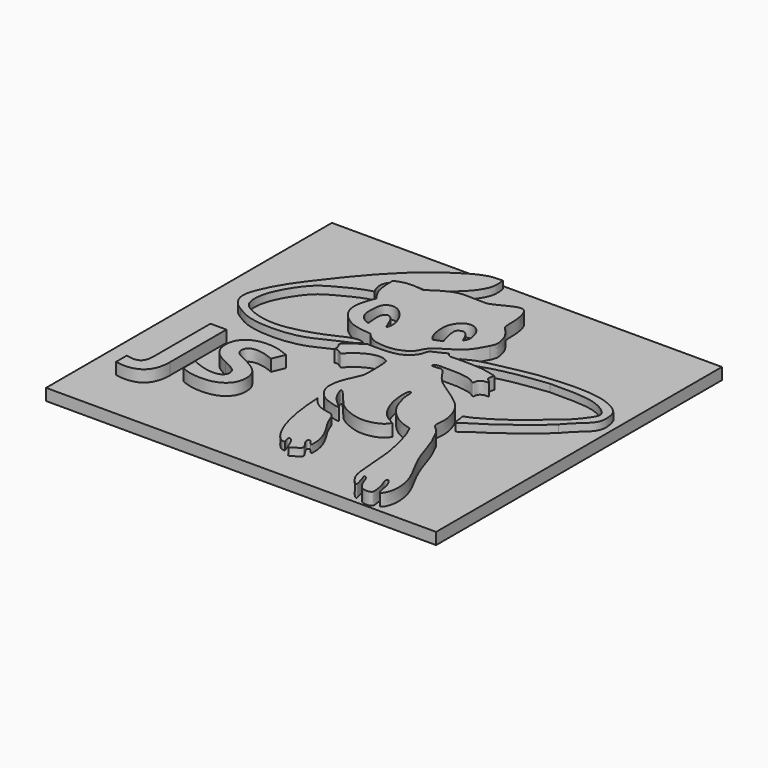
from build123d import *

# Parameters (mm, degrees)
F1_DEPTH     = 5.334
F2_DEPTH     = 3.302
F3_W         = 169.9430719018
F3_H         = 155.6462794542
F4_DEPTH     = 5.08
F5_DEPTH     = 5.08
F6_TEXT_SIZE = 45.9216496286
F7_DEPTH     = 5.08


# Not quite as in the source:
# - Text() gives the source's letters only with a copy of the font that has no kerning and outlines rounded to 1/6400 em; it was checked with that copy


with BuildPart() as f1:
    # F0 (on Top) → F1 (new body)
    with BuildSketch(Plane.XY):
        with BuildLine():
            add(Edge.make_bspline(
                [(-36.8846021593, 36.0807068646), (-37.3919205691, 36.745355779), (-38.573167318, 38.2929329101), (-40.5014475338, 42.4143572996), (-40.7107590613, 48.2182279222), (-40.6138391704, 49.4369952817), (-40.5808985233, 49.8512238264)],
                knots=[0, 0, 0, 0, 0.2194056509, 0.5108669562, 0.8337559114, 1, 1, 1, 1], degree=3))
            add(Edge.make_bspline(
                [(-22.3644245416, 14.6438442171), (-24.6713467296, 14.8439032159), (-29.1783533156, 15.2347561151), (-34.882181479, 17.9727219406), (-39.1312315637, 23.0647945356), (-39.4935763136, 28.8302862551), (-37.8267011281, 33.815991482), (-37.1553457104, 35.4298653868), (-36.8846021593, 36.0807068646)],
                knots=[0, 0, 0, 0, 0.1893684443, 0.3699668893, 0.5515158216, 0.7238806595, 0.8886468645, 1, 1, 1, 1], degree=3))
            add(Edge.make_bspline(
                [(-5.2082133479, 12.2014991939), (-6.1207744444, 11.7172463933), (-8.3286563669, 10.545628396), (-15.353587418, 10.2966075507), (-19.699613734, 11.8971410348), (-21.5102479887, 13.7634179409), (-22.3644245416, 14.6438442171)],
                knots=[0, 0, 0, 0, 0.2165971456, 0.5240426358, 0.775464526, 1, 1, 1, 1], degree=3))
            add(Edge.make_bspline(
                [(15.1303568855, 32.9696908593), (14.5352451306, 31.8316959723), (13.2486953483, 29.3715075085), (10.2455123386, 24.8910940387), (3.5467707647, 21.2909451139), (-0.1632139181, 18.6569829706), (-1.6228436975, 15.6766034686), (-3.1877963332, 12.9531999529), (-4.5795045255, 12.4354117454), (-5.2082133479, 12.2014991939)],
                knots=[0, 0, 0, 0, 0.1407144931, 0.3042053849, 0.4994170574, 0.6491627195, 0.7763538673, 0.8989671128, 1, 1, 1, 1], degree=3))
            add(Edge.make_bspline(
                [(-28.5498145968, 50.8658960462), (-27.3946017427, 51.6630685406), (-24.9466228795, 53.3523342114), (-20.0833499164, 56.0652919109), (-16.3542778469, 56.9634408184), (-12.2867311767, 56.8716252918), (-6.9153223537, 56.7342359886), (-4.3946916269, 56.665054576), (1.0627636823, 59.6982249817), (4.5886739884, 61.236413898), (8.2470343675, 61.4891197316), (9.8575595266, 56.0097175618), (10.1904654801, 52.4142595185), (10.0843781414, 47.0754303269), (11.5893851176, 45.8127835913), (14.8613176101, 41.8496715208), (15.5576528197, 39.0147495294), (16.4135900587, 35.7580508966), (15.5545549064, 33.8914382347), (15.1303568855, 32.9696908593)],
                knots=[0, 0, 0, 0, 0.0621112649, 0.1316182234, 0.188871196, 0.2491962953, 0.3167553376, 0.3643401957, 0.436758445, 0.4967888689, 0.546791506, 0.6123099758, 0.6728165948, 0.7378250462, 0.7790399568, 0.8445049968, 0.8965058511, 0.9488938107, 1, 1, 1, 1], degree=3))
            add(Edge.make_bspline(
                [(-40.5808985233, 49.8512238264), (-39.7577733728, 50.1889108848), (-38.0437485114, 50.8920895121), (-34.9342862767, 51.5058179945), (-31.3792002355, 51.3783823788), (-29.458277106, 51.0304457679), (-28.5498145968, 50.8658960462)],
                knots=[0, 0, 0, 0, 0.234957575, 0.4892611102, 0.7584561682, 1, 1, 1, 1], degree=3))
        make_face()
        with BuildLine():
            add(Edge.make_bspline(
                [(-27.7441535145, 20.2597975731), (-27.836523165, 21.3377254697), (-28.0205851584, 23.4856772729), (-28.2064858053, 26.7533419634), (-27.3095138698, 28.5803581568), (-25.8242693753, 29.158776732), (-23.9397520395, 27.8647529376), (-22.7818146955, 25.7716562911), (-21.7167721967, 22.9536226595), (-21.1669852724, 21.9621876443), (-20.9360662848, 21.5457696468)],
                knots=[0, 0, 0, 0, 0.1498442019, 0.2985896596, 0.4110847443, 0.5056814579, 0.6233821967, 0.7537217582, 0.89655934, 1, 1, 1, 1], degree=3))
            add(Edge.make_bspline(
                [(-20.9360662848, 21.5457696468), (-20.6845803928, 22.4517973521), (-20.1286034759, 24.4548142458), (-21.2599441765, 28.7542103146), (-23.5058865444, 32.3709839432), (-26.9334066004, 35.3160516517), (-30.5123126311, 35.2735079139), (-32.7990191763, 33.0795235548), (-32.9444978647, 29.4825750713), (-33.2245472294, 25.7467879432), (-31.8503260445, 22.5933797005), (-29.5656235756, 20.8892744088), (-28.312173584, 20.4560980688), (-27.7441535145, 20.2597975731)],
                knots=[0, 0, 0, 0, 0.0851228406, 0.1881868366, 0.292340602, 0.3959368999, 0.4853122137, 0.5684365665, 0.6615536453, 0.7584972412, 0.8490847261, 0.9316104312, 1, 1, 1, 1], degree=3))
        make_face(mode=Mode.SUBTRACT)
        with BuildLine():
            add(Edge.make_bspline(
                [(5.4089953192, 30.3651615977), (4.9974793972, 31.3635089709), (4.2164206085, 33.2583760916), (2.492858238, 35.4574563274), (1.1828097347, 35.7536675932), (-1.0889632523, 34.9032052933), (-1.0761434624, 32.5663825666), (-0.7105408655, 30.3909840554), (-0.0619549295, 27.5454399373), (0.4242136144, 26.3185378529), (0.6415589014, 25.7700420916)],
                knots=[0, 0, 0, 0, 0.1500445323, 0.2847850944, 0.377641595, 0.497182947, 0.616278328, 0.7433829902, 0.8852774448, 1, 1, 1, 1], degree=3))
            Line((0.6415589014, 25.7700420916), (-3.0919760466, 24.3340656161))
            add(Edge.make_bspline(
                [(-3.0919760466, 24.3340656161), (-3.6746172439, 25.0952157056), (-4.9790959932, 26.7993590469), (-5.9269204187, 31.3877090281), (-5.8129309399, 36.1864843136), (-3.2806174064, 39.831657957), (-1.0494876922, 41.0503171402), (2.1831388461, 41.2713590695), (5.273039036, 38.380179271), (6.3476776556, 34.9097936113), (6.6819460197, 32.0494739818), (5.8108081984, 30.8968227282), (5.4089953192, 30.3651615977)],
                knots=[0, 0, 0, 0, 0.0943242152, 0.2111830315, 0.3310976043, 0.4422336843, 0.5274260332, 0.6207101402, 0.729021317, 0.8337202238, 0.9233033465, 1, 1, 1, 1], degree=3))
        make_face(mode=Mode.SUBTRACT)
    extrude(amount=F1_DEPTH)


with BuildPart() as f1b:
    # F0 (on Top) → F1, piece 2 (new body)
    with BuildSketch(Plane.XY):
        with BuildLine():
            add(Edge.make_bspline(
                [(30.0683174282, 16.6960265487), (27.7743567444, 17.2982553033), (22.996366427, 18.5526112206), (14.1217566151, 18.5069548483), (10.9595550033, 18.4055071495), (8.914888562, 18.2892193751), (8.1286790312, 19.3965578852), (7.7262688428, 19.9633333832)],
                knots=[0, 0, 0, 0, 0.2687230853, 0.5597115543, 0.7341470669, 0.8639269499, 1, 1, 1, 1], degree=3))
            add(Edge.make_bspline(
                [(7.7262688428, 19.9633333832), (6.7843841918, 19.4219987594), (4.8626373132, 18.3175024471), (0.9491517041, 16.983214183), (0.9172062675, 14.0816922981), (-1.1563972414, 11.1645043961), (-4.2681909188, 8.7975654115), (-10.2481427233, 7.7101704983), (-15.7637806819, 7.8784264398), (-17.5742383687, 7.9638167156), (-18.2920843363, 7.9976739362)],
                knots=[0, 0, 0, 0, 0.1189762035, 0.2427496271, 0.3446266716, 0.463365679, 0.5892044553, 0.7483578638, 0.9002239632, 1, 1, 1, 1], degree=3))
            add(Edge.make_bspline(
                [(-18.2920843363, 7.9976739362), (-19.2081909322, 7.3508545619), (-21.220968544, 5.9297278487), (-26.2844384077, 2.5837754081), (-25.5818429798, 1.1641009834), (-24.788360107, 0.7943681377), (-24.7400624967, -0.7928668879), (-24.7462409395, -1.4706101124), (-24.7490536422, -1.7791490536)],
                knots=[0, 0, 0, 0, 0.2335516694, 0.5131363244, 0.6318283516, 0.7367278182, 0.8801467617, 1, 1, 1, 1], degree=3))
            add(Edge.make_bspline(
                [(-24.7490536422, -1.7791490536), (-24.2594300604, -1.6489843167), (-23.1371940302, -1.3506417469), (-20.7418558435, -3.9319628807), (-19.8396284785, -1.3153314822), (-15.2791573927, 1.747858691), (-12.0049756273, 3.1979621252), (-8.2035408147, 3.7607412239), (-6.3214470372, 2.7044753683), (-5.4122591391, 2.1942222957)],
                knots=[0, 0, 0, 0, 0.1027998361, 0.2356211674, 0.3469371625, 0.5398555958, 0.7001501422, 0.8551507554, 1, 1, 1, 1], degree=3))
            add(Edge.make_bspline(
                [(-5.4122591391, -11.4604206756), (-5.2622117063, -11.0833952824), (-4.8483954868, -10.0435959346), (-4.8531432648, -5.796717989), (-4.8905091249, -0.455510217), (-5.2613557919, 1.4278523975), (-5.4122591391, 2.1942222957)],
                knots=[0, 0, 0, 0, 0.16298087, 0.4494853805, 0.7759869344, 1, 1, 1, 1], degree=3))
            add(Edge.make_bspline(
                [(-5.4122591391, -11.4604206756), (-5.7180365241, -12.1910633261), (-6.4589745929, -13.9615047682), (-8.7341618296, -18.823732403), (-9.3339817846, -22.6702412315), (-9.3862087635, -25.4827799286), (-8.6161951623, -27.2256408895), (-8.2267019898, -28.1072258949)],
                knots=[0, 0, 0, 0, 0.1760181488, 0.4265146922, 0.6415927054, 0.8187081449, 1, 1, 1, 1], degree=3))
            add(Edge.make_bspline(
                [(-8.2267019898, -28.1072258949), (-7.6234509095, -28.9847780463), (-6.3158368471, -30.886970303), (-3.3578440432, -33.0385452557), (4.7605685311, -35.3009211391), (0.7062696421, -32.348079143), (-2.6369370543, -28.938166705), (-4.7745965374, -23.008879984), (-2.1692361288, -25.4214104232), (0.0596427785, -28.1204059957), (3.5703763797, -32.828689266), (9.4441591128, -35.6788887604), (15.6783436568, -37.2193911759), (22.840726257, -35.0789922839), (24.1300062291, -32.9878270093), (24.6503651142, -32.1438238025)],
                knots=[0, 0, 0, 0, 0.0644771481, 0.1397614166, 0.2278212025, 0.2838940026, 0.3731896446, 0.4478304981, 0.4963143315, 0.5679076052, 0.6548180235, 0.7466462144, 0.8393730298, 0.9351702711, 1, 1, 1, 1], degree=3))
            add(Edge.make_bspline(
                [(24.6503651142, -32.1438238025), (22.7874017729, -31.1547850766), (18.978892069, -29.1328646762), (15.7565133464, -22.5588668197), (14.3110475227, -17.0219112758), (14.2258983476, -9.955668629), (16.1051306441, -10.5144580218), (15.6702473707, -13.747750159), (17.0855807883, -18.568062254), (18.3355817835, -22.1596484216), (21.6146077655, -26.502386498), (26.1560860605, -29.9186464967), (29.8500456849, -30.9730548373), (31.7023843527, -31.501788646)],
                knots=[0, 0, 0, 0, 0.1044502141, 0.213530586, 0.3203453584, 0.4213187613, 0.4580269744, 0.5290816996, 0.6236498562, 0.7054940824, 0.8011178875, 0.9002704239, 1, 1, 1, 1], degree=3))
            add(Edge.make_bspline(
                [(31.7023843527, -31.501788646), (32.4317515175, -33.0339186757), (34.0418847304, -36.4162116639), (35.891222752, -44.0199699231), (36.7066142268, -48.1595329342), (36.9354538826, -49.5206387254), (37.0256751776, -50.0572621822)],
                knots=[0, 0, 0, 0, 0.2736015544, 0.6039961368, 0.8438732953, 1, 1, 1, 1], degree=3))
            add(Edge.make_bspline(
                [(37.0256751776, -50.0572621822), (37.2529570378, -52.2585996466), (37.7295250837, -56.874397374), (38.1744288141, -65.147375762), (39.0614282703, -71.473936135), (43.7073747885, -75.9926535392), (43.0041439625, -73.1870722683), (42.5863736095, -71.2442159702), (41.2192631142, -68.0900104475), (43.2122596535, -69.062811459), (43.8660534195, -72.1091856839), (46.0001837404, -75.8667367907), (48.2415322815, -76.7510536361), (51.5666329574, -76.464046498), (51.0718324014, -73.597450229), (50.7537782092, -69.9651897279), (49.0133489818, -67.3461961901), (49.5300726584, -65.1991280143), (51.3610203699, -67.2721869465), (52.3453968623, -70.4529473283), (52.995619021, -76.2204950553), (56.059449066, -71.996615036), (56.1941191956, -64.2541648711), (53.057015864, -56.2370554706), (47.5422537848, -47.2864849217), (44.2428025956, -35.181683009), (42.4634124655, -31.9627538165), (41.779063642, -30.7247620076)],
                knots=[0, 0, 0, 0, 0.0515181447, 0.1080240258, 0.1600193281, 0.200966199, 0.2242692528, 0.2561913518, 0.2869292175, 0.3071601688, 0.3426397052, 0.3829711635, 0.4133879878, 0.44506026, 0.4747807776, 0.5132716918, 0.5483859123, 0.5705941331, 0.5969574393, 0.6366393869, 0.6760617143, 0.7097084145, 0.7649651301, 0.8224062602, 0.8873011559, 0.9566563172, 1, 1, 1, 1], degree=3))
            add(Edge.make_bspline(
                [(41.779063642, -30.7247620076), (41.220519955, -29.4131194944), (40.1405083976, -26.8769005623), (36.3496730282, -24.6391556022), (37.9091307315, -19.6176807334), (35.5635143336, -10.6479929739), (30.5388392719, -5.8669855098), (23.9637593307, -1.3236326178), (17.1210038146, 2.9501551711), (13.8645399549, 9.8095100123), (11.3218741684, 9.2331700055), (8.0189997491, 8.9048258219), (9.6884536448, 10.9398859033), (12.9400373278, 10.6519892488), (17.7385160156, 10.8919830294), (21.7909115084, 10.3524706804), (25.1173197763, 9.8387273821), (27.8544362389, 7.7039501469), (27.5140398783, 10.0552824679), (29.4509197324, 11.6524955754), (32.6539040013, 11.3234634506), (30.9452406108, 12.542717614), (30.0683174282, 13.1684653461)],
                knots=[0, 0, 0, 0, 0.0519267935, 0.1004067156, 0.1547860225, 0.2308120849, 0.2975658467, 0.3688932812, 0.4426002883, 0.5078563984, 0.5467057553, 0.5855180915, 0.6152135834, 0.6611250141, 0.7174470552, 0.7689076739, 0.8172224822, 0.8564603738, 0.8862383123, 0.9262880687, 0.962169435, 1, 1, 1, 1], degree=3))
            add(Edge.make_bspline(
                [(30.0683174282, 13.1684653461), (29.9041852058, 13.3684306238), (29.4381629957, 13.9361939752), (29.8205842702, 15.6110511778), (30.0683174282, 16.6960265487)],
                knots=[0, 0, 0, 0, 0.3521982834, 1, 1, 1, 1], degree=3))
        make_face()
    extrude(amount=F1_DEPTH)


with BuildPart() as f2:
    # F0 (on Top) → F2 (new body)
    with BuildSketch(Plane.XY):
        with BuildLine():
            add(Edge.make_bspline(
                [(-43.0377721786, 42.7853837609), (-43.4217519294, 43.5555106027), (-44.2704707094, 45.2577386818), (-44.7495303082, 49.6843935754), (-41.0137641329, 52.7815034964), (-36.6859509281, 54.4525017318), (-31.3441059726, 54.4142323895), (-29.2217337248, 54.0177284331), (-28.3044036478, 53.8463518023)],
                knots=[0, 0, 0, 0, 0.1383428068, 0.3057821096, 0.4812834692, 0.6632360629, 0.8544441539, 1, 1, 1, 1], degree=3))
            add(Edge.make_bspline(
                [(-28.3044036478, 53.8463518023), (-26.4073160355, 55.6555092544), (-22.6771829073, 59.2127504184), (-17.2353435255, 63.8393788129), (-13.8276032853, 69.6509731284), (-13.5447997553, 73.3805690433), (-13.8346112059, 75.3733824514), (-13.9714321122, 76.3141959906)],
                knots=[0, 0, 0, 0, 0.2399087284, 0.471718591, 0.6909669262, 0.8541045044, 1, 1, 1, 1], degree=3))
            add(Edge.make_bspline(
                [(-13.9714321122, 76.3141959906), (-15.6695767931, 76.3303285057), (-19.2883266624, 76.3647069291), (-25.3938334761, 73.7499379423), (-32.2227465198, 69.3257394868), (-37.0027510136, 65.6788461869), (-41.5089383745, 61.9702597728), (-43.2950078592, 60.2558688539), (-44.0782904625, 59.5040209591)],
                knots=[0, 0, 0, 0, 0.1571726677, 0.3349352838, 0.5326783847, 0.7051580212, 0.870696748, 1, 1, 1, 1], degree=3))
            add(Edge.make_bspline(
                [(-44.0782904625, 59.5040209591), (-46.5278412391, 57.082066591), (-52.097162839, 51.575488444), (-63.3309865981, 37.4942248425), (-71.4221468374, 26.4624379543), (-75.7339498561, 17.0106297705), (-76.6395144361, 11.8788318896), (-75.1074330935, 8.3160305556), (-73.204783322, 6.068043111), (-71.7088671371, 5.0905988199), (-70.9798410535, 4.6142470092)],
                knots=[0, 0, 0, 0, 0.1518529739, 0.3452543444, 0.517129726, 0.6613859031, 0.7623466126, 0.8489157512, 0.9263699669, 1, 1, 1, 1], degree=3))
            add(Edge.make_bspline(
                [(-70.9798410535, 4.6142470092), (-69.3666307118, 3.5770845145), (-65.6901376032, 1.2133997143), (-55.8893542983, -0.5183749), (-41.2432784113, 0.4464145968), (-31.0706871572, 6.483604405), (-24.0806480786, 8.8396956503), (-21.752412637, 11.3394508322), (-26.5347743619, 12.1529097756), (-32.3033005496, 9.1331545972), (-40.0565385081, 5.9205974959), (-50.0430210503, 3.1697487317), (-58.8129954214, 2.9178477888), (-66.9351159188, 5.4707126725), (-72.0186295298, 9.156570048), (-71.6690554507, 18.4329778003), (-66.5327096092, 27.8683616368), (-61.2862876559, 34.4220241119), (-54.7268271319, 37.7283730842), (-48.6744931046, 41.0395084453), (-44.8645902562, 42.2195589437), (-43.0377721786, 42.7853837609)],
                knots=[0, 0, 0, 0, 0.0465524502, 0.1060926513, 0.1790243597, 0.2452061951, 0.2968084881, 0.3232171179, 0.357646466, 0.4069920351, 0.4626730308, 0.5238603294, 0.5805035455, 0.6354123547, 0.6802029703, 0.7351769542, 0.7981924539, 0.8529702112, 0.9040331392, 0.9539846544, 1, 1, 1, 1], degree=3))
        make_face()
    extrude(amount=F2_DEPTH)


with BuildPart() as f2b:
    # F0 (on Top) → F2, piece 2 (new body)
    with BuildSketch(Plane.XY):
        with BuildLine():
            add(Edge.make_bspline(
                [(2.3568598554, -62.7967566252), (1.849591697, -62.7900183143), (0.4679465245, -62.7716651917), (-3.2310828631, -58.8113433278), (-6.7057614708, -50.0665204215), (-8.6370836456, -38.8411168477), (-8.9614558541, -33.2628901217), (-9.1090472415, -30.7247620076)],
                knots=[0, 0, 0, 0, 0.099509161, 0.2710328838, 0.51388907, 0.7788164808, 1, 1, 1, 1], degree=3))
            add(Edge.make_bspline(
                [(-9.1090472415, -30.7247620076), (-8.4235955574, -31.6189211927), (-6.9475052353, -33.5444540203), (-3.101528472, -36.1875069597), (1.8982272323, -36.366099626), (3.4405558722, -38.6877901024), (4.4761606927, -42.3593420867), (7.8964967826, -47.1650437774), (10.103858215, -52.0425869753), (10.7860608645, -55.6476684863), (10.6753618785, -57.5461375395), (10.9225050319, -59.3049638311), (9.4107167153, -57.6424469164), (8.5616404275, -56.4503239427), (7.5237963592, -56.8148042208), (7.6117730332, -58.1583165289), (8.9359028975, -60.1929547878), (10.1219675513, -61.7535687362), (9.4773292634, -62.9623853428), (7.0627564007, -64.3325582518), (5.4694748144, -65.4986569004), (4.5573424059, -62.78355908), (3.3761804254, -60.4551449839), (2.1377112045, -59.3756823228), (1.4345728768, -60.1256467658), (1.8841051195, -61.4401596052), (2.1958233582, -62.3346530955), (2.3568598554, -62.7967566252)],
                knots=[0, 0, 0, 0, 0.0496809561, 0.1069857733, 0.1646060762, 0.2058387605, 0.2571628324, 0.3222353289, 0.3845712685, 0.4346179158, 0.4726711954, 0.4992092936, 0.5325676268, 0.5654673868, 0.5880449987, 0.6160765379, 0.6586074123, 0.6943476006, 0.72222254, 0.7675356615, 0.7994953394, 0.8396297218, 0.8851573032, 0.9154600181, 0.9370908196, 0.9675005412, 1, 1, 1, 1], degree=3))
        make_face()
    extrude(amount=F2_DEPTH)


with BuildPart() as f2c:
    # F0 (on Top) → F2, piece 3 (new body)
    with BuildSketch(Plane.XY):
        with BuildLine():
            add(Edge.make_bspline(
                [(10.7216527686, 22.0162756741), (12.1246687267, 22.8148610446), (15.339687331, 24.6448237106), (23.6197362006, 26.4763189676), (32.72292454, 28.3516074967), (37.0192507628, 29.0816873989), (38.9400422573, 29.4080898166)],
                knots=[0, 0, 0, 0, 0.210423914, 0.4821875291, 0.7684976098, 1, 1, 1, 1], degree=3))
            add(Edge.make_bspline(
                [(10.7216527686, 22.0162756741), (11.0952281861, 21.6401005628), (11.9676852339, 20.7615721278), (15.1851161792, 20.2060896425), (20.1867499974, 22.1900920896), (27.3159099422, 24.2389696372), (36.615664636, 25.8884813304), (42.8756191809, 26.6520064029), (46.0081286728, 27.0340777934)],
                knots=[0, 0, 0, 0, 0.0904593315, 0.2112609063, 0.3729533578, 0.5659140772, 0.7827814461, 1, 1, 1, 1], degree=3))
            add(Edge.make_bspline(
                [(46.0081286728, 27.0340777934), (48.7258841079, 27.0612678355), (54.4256706903, 27.1182918912), (64.5466285691, 26.6819854244), (71.2784960569, 23.5683344076), (74.4956568823, 20.0928312055), (72.370302212, 16.1583995878), (68.2328509473, 10.8727360954), (63.0282482519, 6.6939099868), (60.288196872, 4.4211072069), (59.0115785599, 3.3621848561)],
                knots=[0, 0, 0, 0, 0.1437483771, 0.3014749084, 0.4359008913, 0.5332154076, 0.6294905174, 0.7592457502, 0.8878301019, 1, 1, 1, 1], degree=3))
            add(Edge.make_bspline(
                [(59.0115785599, 3.3621848561), (56.9423383347, 1.6375621217), (52.775286197, -1.8354966196), (46.5278179073, -6.1349616625), (39.331175356, -10.0891007633), (37.5946538004, -10.0778540145), (38.361869053, -11.9948167923), (38.4145231293, -16.8707660308), (41.9490027911, -13.083803004), (47.7757044759, -10.0981764978), (54.0702257822, -5.0810900312), (60.5319653238, -0.5910086566), (64.8441388463, 3.4273348996), (67.067630589, 5.4993187077)],
                knots=[0, 0, 0, 0, 0.1094389502, 0.2203890133, 0.3295663194, 0.369726266, 0.4213415268, 0.4936271411, 0.5627007536, 0.6656686645, 0.7754420094, 0.884210866, 1, 1, 1, 1], degree=3))
            add(Edge.make_bspline(
                [(67.067630589, 5.4993187077), (68.4073962182, 7.0026565142), (71.2661439341, 10.3161375403), (78.3602736598, 15.59597471), (76.7631828785, 22.33495377), (75.9328380227, 24.1133533418)],
                knots=[0, 0, 0, 0, 0.3098887474, 0.6604961476, 1, 1, 1, 1], degree=3))
            add(Edge.make_bspline(
                [(38.9400422573, 29.4080898166), (42.1234440462, 29.7199891996), (48.5724313187, 30.3518400576), (58.6475201749, 30.6661036157), (67.9584350083, 29.3917039016), (73.8641097497, 26.3531807622), (75.3402605954, 24.7549413105), (75.9328380227, 24.1133533418)],
                knots=[0, 0, 0, 0, 0.2286564396, 0.4632159453, 0.6902384315, 0.8756511139, 1, 1, 1, 1], degree=3))
        make_face()
    extrude(amount=F2_DEPTH)


with BuildPart() as f4:
    # F3 (on face) → F4 (new body)
    with BuildSketch(Plane(origin=(0, 0, 0), x_dir=(1, 0, 0), z_dir=(0, 0, -1))):
        with Locations((-4.9392692745, -0.3463253379)):
            Rectangle(F3_W, F3_H)
        with BuildLine():
            add(Edge.make_bspline(
                [(30.0683174282, -13.1684653461), (29.9041852058, -13.3684306238), (29.4381629957, -13.9361939752), (29.8205842702, -15.6110511778), (30.0683174282, -16.6960265487)],
                knots=[0, 0, 0, 0, 0.3521982834, 1, 1, 1, 1], degree=3))
            add(Edge.make_bspline(
                [(30.0683174282, -16.6960265487), (27.7743567444, -17.2982553033), (22.996366427, -18.5526112206), (14.1217566151, -18.5069548483), (10.9595550033, -18.4055071495), (8.914888562, -18.2892193751), (8.1286790312, -19.3965578852), (7.7262688428, -19.9633333832)],
                knots=[0, 0, 0, 0, 0.2687230853, 0.5597115543, 0.7341470669, 0.8639269499, 1, 1, 1, 1], degree=3))
            add(Edge.make_bspline(
                [(7.7262688428, -19.9633333832), (6.7843841918, -19.4219987594), (4.8626373132, -18.3175024471), (0.9491517041, -16.983214183), (0.9172062675, -14.0816922981), (-1.1563972414, -11.1645043961), (-4.2681909188, -8.7975654115), (-10.2481427233, -7.7101704983), (-15.7637806819, -7.8784264398), (-17.5742383687, -7.9638167156), (-18.2920843363, -7.9976739362)],
                knots=[0, 0, 0, 0, 0.1189762035, 0.2427496271, 0.3446266716, 0.463365679, 0.5892044553, 0.7483578638, 0.9002239632, 1, 1, 1, 1], degree=3))
            add(Edge.make_bspline(
                [(-18.2920843363, -7.9976739362), (-19.2081909322, -7.3508545619), (-21.220968544, -5.9297278487), (-26.2844384077, -2.5837754081), (-25.5818429798, -1.1641009834), (-24.788360107, -0.7943681377), (-24.7400624967, 0.7928668879), (-24.7462409395, 1.4706101124), (-24.7490536422, 1.7791490536)],
                knots=[0, 0, 0, 0, 0.2335516694, 0.5131363244, 0.6318283516, 0.7367278182, 0.8801467617, 1, 1, 1, 1], degree=3))
            add(Edge.make_bspline(
                [(-24.7490536422, 1.7791490536), (-24.2594300604, 1.6489843167), (-23.1371940302, 1.3506417469), (-20.7418558435, 3.9319628807), (-19.8396284785, 1.3153314822), (-15.2791573927, -1.747858691), (-12.0049756273, -3.1979621252), (-8.2035408147, -3.7607412239), (-6.3214470372, -2.7044753683), (-5.4122591391, -2.1942222957)],
                knots=[0, 0, 0, 0, 0.1027998361, 0.2356211674, 0.3469371625, 0.5398555958, 0.7001501422, 0.8551507554, 1, 1, 1, 1], degree=3))
            add(Edge.make_bspline(
                [(-5.4122591391, 11.4604206756), (-5.2622117063, 11.0833952824), (-4.8483954868, 10.0435959346), (-4.8531432648, 5.796717989), (-4.8905091249, 0.455510217), (-5.2613557919, -1.4278523975), (-5.4122591391, -2.1942222957)],
                knots=[0, 0, 0, 0, 0.16298087, 0.4494853805, 0.7759869344, 1, 1, 1, 1], degree=3))
            add(Edge.make_bspline(
                [(-5.4122591391, 11.4604206756), (-5.7180365241, 12.1910633261), (-6.4589745929, 13.9615047682), (-8.7341618296, 18.823732403), (-9.3339817846, 22.6702412315), (-9.3862087635, 25.4827799286), (-8.6161951623, 27.2256408895), (-8.2267019898, 28.1072258949)],
                knots=[0, 0, 0, 0, 0.1760181488, 0.4265146922, 0.6415927054, 0.8187081449, 1, 1, 1, 1], degree=3))
            add(Edge.make_bspline(
                [(-8.2267019898, 28.1072258949), (-7.6234509095, 28.9847780463), (-6.3158368471, 30.886970303), (-3.3578440432, 33.0385452557), (4.7605685311, 35.3009211391), (0.7062696421, 32.348079143), (-2.6369370543, 28.938166705), (-4.7745965374, 23.008879984), (-2.1692361288, 25.4214104232), (0.0596427785, 28.1204059957), (3.5703763797, 32.828689266), (9.4441591128, 35.6788887604), (15.6783436568, 37.2193911759), (22.840726257, 35.0789922839), (24.1300062291, 32.9878270093), (24.6503651142, 32.1438238025)],
                knots=[0, 0, 0, 0, 0.0644771481, 0.1397614166, 0.2278212025, 0.2838940026, 0.3731896446, 0.4478304981, 0.4963143315, 0.5679076052, 0.6548180235, 0.7466462144, 0.8393730298, 0.9351702711, 1, 1, 1, 1], degree=3))
            add(Edge.make_bspline(
                [(24.6503651142, 32.1438238025), (22.7874017729, 31.1547850766), (18.978892069, 29.1328646762), (15.7565133464, 22.5588668197), (14.3110475227, 17.0219112758), (14.2258983476, 9.955668629), (16.1051306441, 10.5144580218), (15.6702473707, 13.747750159), (17.0855807883, 18.568062254), (18.3355817835, 22.1596484216), (21.6146077655, 26.502386498), (26.1560860605, 29.9186464967), (29.8500456849, 30.9730548373), (31.7023843527, 31.501788646)],
                knots=[0, 0, 0, 0, 0.1044502141, 0.213530586, 0.3203453584, 0.4213187613, 0.4580269744, 0.5290816996, 0.6236498562, 0.7054940824, 0.8011178875, 0.9002704239, 1, 1, 1, 1], degree=3))
            add(Edge.make_bspline(
                [(31.7023843527, 31.501788646), (32.4317515175, 33.0339186757), (34.0418847304, 36.4162116639), (35.891222752, 44.0199699231), (36.7066142268, 48.1595329342), (36.9354538826, 49.5206387254), (37.0256751776, 50.0572621822)],
                knots=[0, 0, 0, 0, 0.2736015544, 0.6039961368, 0.8438732953, 1, 1, 1, 1], degree=3))
            add(Edge.make_bspline(
                [(37.0256751776, 50.0572621822), (37.2529570378, 52.2585996466), (37.7295250837, 56.874397374), (38.1744288141, 65.147375762), (39.0614282703, 71.473936135), (43.7073747885, 75.9926535392), (43.0041439625, 73.1870722683), (42.5863736095, 71.2442159702), (41.2192631142, 68.0900104475), (43.2122596535, 69.062811459), (43.8660534195, 72.1091856839), (46.0001837404, 75.8667367907), (48.2415322815, 76.7510536361), (51.5666329574, 76.464046498), (51.0718324014, 73.597450229), (50.7537782092, 69.9651897279), (49.0133489818, 67.3461961901), (49.5300726584, 65.1991280143), (51.3610203699, 67.2721869465), (52.3453968623, 70.4529473283), (52.995619021, 76.2204950553), (56.059449066, 71.996615036), (56.1941191956, 64.2541648711), (53.057015864, 56.2370554706), (47.5422537848, 47.2864849217), (44.2428025956, 35.181683009), (42.4634124655, 31.9627538165), (41.779063642, 30.7247620076)],
                knots=[0, 0, 0, 0, 0.0515181447, 0.1080240258, 0.1600193281, 0.200966199, 0.2242692528, 0.2561913518, 0.2869292175, 0.3071601688, 0.3426397052, 0.3829711635, 0.4133879878, 0.44506026, 0.4747807776, 0.5132716918, 0.5483859123, 0.5705941331, 0.5969574393, 0.6366393869, 0.6760617143, 0.7097084145, 0.7649651301, 0.8224062602, 0.8873011559, 0.9566563172, 1, 1, 1, 1], degree=3))
            add(Edge.make_bspline(
                [(41.779063642, 30.7247620076), (41.220519955, 29.4131194944), (40.1405083976, 26.8769005623), (36.3496730282, 24.6391556022), (37.9091307315, 19.6176807334), (35.5635143336, 10.6479929739), (30.5388392719, 5.8669855098), (23.9637593307, 1.3236326178), (17.1210038146, -2.9501551711), (13.8645399549, -9.8095100123), (11.3218741684, -9.2331700055), (8.0189997491, -8.9048258219), (9.6884536448, -10.9398859033), (12.9400373278, -10.6519892488), (17.7385160156, -10.8919830294), (21.7909115084, -10.3524706804), (25.1173197763, -9.8387273821), (27.8544362389, -7.7039501469), (27.5140398783, -10.0552824679), (29.4509197324, -11.6524955754), (32.6539040013, -11.3234634506), (30.9452406108, -12.542717614), (30.0683174282, -13.1684653461)],
                knots=[0, 0, 0, 0, 0.0519267935, 0.1004067156, 0.1547860225, 0.2308120849, 0.2975658467, 0.3688932812, 0.4426002883, 0.5078563984, 0.5467057553, 0.5855180915, 0.6152135834, 0.6611250141, 0.7174470552, 0.7689076739, 0.8172224822, 0.8564603738, 0.8862383123, 0.9262880687, 0.962169435, 1, 1, 1, 1], degree=3))
        make_face(mode=Mode.SUBTRACT)
    extrude(amount=F4_DEPTH)

    # F6 (on face) → F7 (join)
    with BuildSketch(Plane.XY):
        with Locations((-73.7823843956, -46.0607819259)):
            Text('JS', F6_TEXT_SIZE, font='Open Sans', font_style=FontStyle.BOLD, text_align=(TextAlign.LEFT, TextAlign.BOTTOM))
    extrude(amount=F7_DEPTH)


with BuildPart() as f5:
    # F5 (new): a face of the model
    f5_faces = [f1b.part.faces().sort_by_distance(p)[0] for p in [
        (18.9065912912, -20.1747019139, 0),
    ]]
    extrude(f5_faces, amount=F5_DEPTH)


solid = Compound([f1.part, f1b.part, f2.part, f2b.part, f2c.part, f4.part, f5.part])
